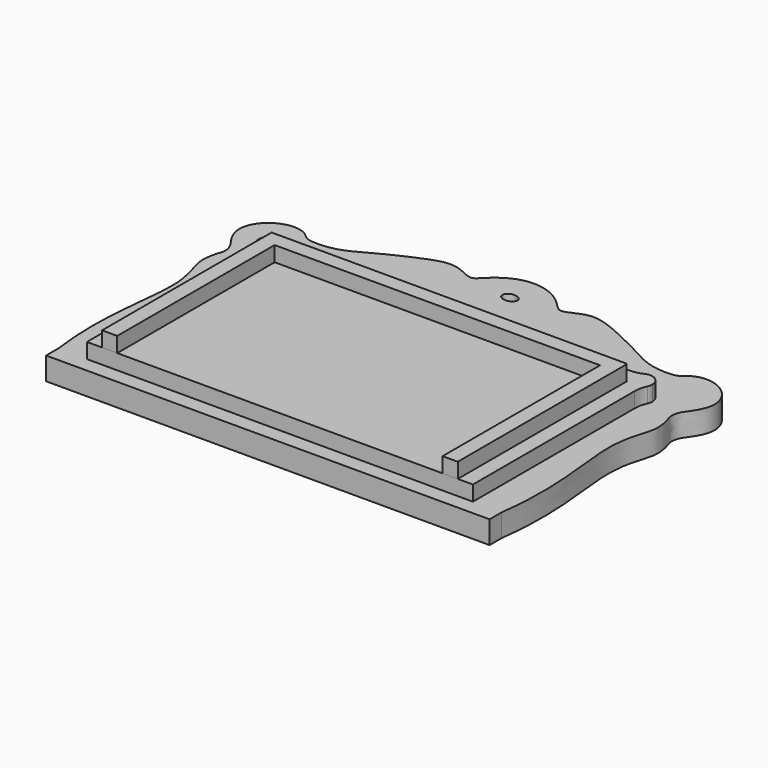
from build123d import *

# Parameters (mm, degrees)
F2_W      = 292.994
F2_H      = 10
F3_DEPTH  = 15
F5_DEPTH  = 10
F6_R      = 20
F8_DEPTH  = 10
F9_W      = 215
F9_H      = 130
F10_DEPTH = 10


# Not quite as in the source:
# - a feature of the source that left no trace in its solid (it failed there, or was rolled back) is left out
# - a feature names something its author has since deleted; it is built from what else it names


with BuildPart() as f3:
    # F2 (on offset) → F3 (new body)
    with BuildSketch(Plane.XY.offset(100)):
        with BuildLine():
            add(Edge.make_bspline(
                [(-146.497, 0), (-149.5984924285, 24.1158641447), (-148.0861706874, 57.3285451295), (-141.9737942158, 98.5465216918), (-150.8716245384, 120.1352309784), (-150.0828583406, 127.8333799004), (-149.2091995607, 133.0357574413), (-146.7644359487, 138.969514697), (-148.7060186985, 145.4416060002), (-153.4320405507, 150.8180485227), (-159.2044434643, 163.229297572), (-152.2232789146, 177.3369452319), (-138.5120912335, 183.3796622376), (-127.657061459, 180.8243319765), (-123.7549340061, 175.7598872143), (-115.4966109213, 174.5749138288), (-101.1868476342, 175.8719474345), (-83.9780063011, 186.2524528593), (-68.1221038647, 193.6100878861), (-57.6143130787, 198.1949467154), (-46.4912789312, 200.9893875839), (-38.3855377787, 198.1650207363), (-34.3252044535, 195.9531038256), (-28.5769681871, 194.0801714579), (-24.8215233637, 198.3952390386), (-15.2356704617, 207.2522812764), (0, 211.4399134414), (15.2356704617, 207.2522812764), (24.8215233637, 198.3952390386), (28.5769681871, 194.0801714579), (34.3252044535, 195.9531038256), (38.3855377787, 198.1650207363), (46.4912789312, 200.9893875839), (57.6143130787, 198.1949467154), (68.1221038647, 193.6100878861), (83.9780063011, 186.2524528593), (101.1868476342, 175.8719474345), (115.4966109213, 174.5749138288), (123.7549340061, 175.7598872143), (127.657061459, 180.8243319765), (138.5120912335, 183.3796622376), (152.2232789146, 177.3369452319), (159.2044434643, 163.229297572), (153.4320405507, 150.8180485227), (148.7060186985, 145.4416060002), (146.7644359487, 138.969514697), (149.2091995607, 133.0357574413), (150.0828583406, 127.8333799004), (150.8716245384, 120.1352309784), (141.9737942158, 98.5465216918), (148.0861706874, 57.3285451295), (149.5984924285, 24.1158641447), (146.497, 0)],
                knots=[0, 0, 0, 0, 0.0445117001, 0.0808774056, 0.107575939, 0.1227793119, 0.1357551155, 0.1500456603, 0.1643362052, 0.1797671231, 0.2002043009, 0.2219477978, 0.2436912948, 0.2620418522, 0.2758571435, 0.2916470183, 0.3132257177, 0.3392061483, 0.3632884541, 0.3827866647, 0.4019539182, 0.4183166408, 0.4309215947, 0.4439460967, 0.456795292, 0.4773590218, 0.5, 0.5226409782, 0.543204708, 0.5560539033, 0.5690784053, 0.5816833592, 0.5980460818, 0.6172133353, 0.6367115459, 0.6607938517, 0.6867742823, 0.7083529817, 0.7241428565, 0.7379581478, 0.7563087052, 0.7780522022, 0.7997956991, 0.8202328769, 0.8356637948, 0.8499543397, 0.8642448845, 0.8772206881, 0.892424061, 0.9191225944, 0.9554882999, 1, 1, 1, 1], degree=3))
            Line((-146.497, 0), (146.497, 0))
        make_face()
        with BuildLine():
            add(Edge.make_bspline(
                [(5, 190), (5, 196.4951905284), (-2.5, 193.2475952642), (-10, 190), (-2.5, 186.7524047358), (5, 183.5048094716), (5, 190)],
                knots=[0, 0, 0, 2.0943951024, 2.0943951024, 4.1887902048, 4.1887902048, 6.2831853072, 6.2831853072, 6.2831853072], degree=2, weights=[1, 0.5, 1, 0.5, 1, 0.5, 1]))
        make_face(mode=Mode.SUBTRACT)
        with Locations((0, -5)):
            Rectangle(F2_W, F2_H)
    extrude(amount=F3_DEPTH)


with BuildPart() as f5:
    # F4 (on face) → F5 (new body)
    with BuildSketch(Plane.XY.offset(115)):
        with BuildLine():
            Line((-116.9098300563, 150), (-127.5, 150))
            Line((-127.5, 150), (-117.5, 140))
            Line((-117.5, 140), (-116.9098300563, 140))
            ThreePointArc((-116.9098300563, 140), (-115.4937073078, 142.3238343267), (-115, 145))
            ThreePointArc((-115, 145), (-115.4937073078, 147.6761656733), (-116.9098300563, 150))
        make_face()
        with BuildLine():
            Line((116.9098300563, 150), (-116.9098300563, 150))
            ThreePointArc((-116.9098300563, 150), (-115.4937073078, 147.6761656733), (-115, 145))
            ThreePointArc((-115, 145), (-115.4937073078, 142.3238343267), (-116.9098300563, 140))
            Line((-116.9098300563, 140), (116.9098300563, 140))
            ThreePointArc((116.9098300563, 140), (115, 145), (116.9098300563, 150))
        make_face()
        with BuildLine():
            Line((117.5, 140), (117.5, 139.4098300563))
            ThreePointArc((117.5, 139.4098300563), (122.5, 137.5), (127.5, 139.4098300563))
            Line((127.5, 139.4098300563), (127.5, 150))
            Line((127.5, 150), (116.9098300563, 150))
            ThreePointArc((116.9098300563, 150), (115, 145), (116.9098300563, 140))
            Line((116.9098300563, 140), (117.5, 140))
        make_face()
        with BuildLine():
            Line((-117.5, 139.4098300563), (-117.5, 0))
            Line((-117.5, 0), (117.5, 0))
            Line((117.5, 0), (117.5, 139.4098300563))
            ThreePointArc((117.5, 139.4098300563), (117.1966991411, 139.6966991411), (116.9098300563, 140))
            Line((116.9098300563, 140), (-116.9098300563, 140))
            ThreePointArc((-116.9098300563, 140), (-117.1966991411, 139.6966991411), (-117.5, 139.4098300563))
        make_face()
        with BuildLine():
            Line((-127.5, 150), (-127.5, 139.4098300563))
            ThreePointArc((-127.5, 139.4098300563), (-122.5, 137.5), (-117.5, 139.4098300563))
            Line((-117.5, 139.4098300563), (-117.5, 140))
            Line((-117.5, 140), (-127.5, 150))
        make_face()
        with BuildLine():
            Line((-117.5, 140), (-117.5, 139.4098300563))
            ThreePointArc((-117.5, 139.4098300563), (-117.1966991411, 139.6966991411), (-116.9098300563, 140))
            Line((-116.9098300563, 140), (-117.5, 140))
        make_face()
        with BuildLine():
            Line((-127.5, 139.4098300563), (-127.5, 0))
            Line((-127.5, 0), (-117.5, 0))
            Line((-117.5, 0), (-117.5, 139.4098300563))
            ThreePointArc((-117.5, 139.4098300563), (-122.5, 137.5), (-127.5, 139.4098300563))
        make_face()
        with BuildLine():
            Line((117.5, 139.4098300563), (117.5, 0))
            Line((117.5, 0), (127.5, 0))
            Line((127.5, 0), (127.5, 139.4098300563))
            ThreePointArc((127.5, 139.4098300563), (122.5, 137.5), (117.5, 139.4098300563))
        make_face()
        with BuildLine():
            ThreePointArc((-116.9098300563, 150), (-127.8033008589, 150.3033008589), (-127.5, 139.4098300563))
            Line((-127.5, 139.4098300563), (-127.5, 150))
            Line((-127.5, 150), (-116.9098300563, 150))
        make_face()
        with BuildLine():
            ThreePointArc((130, 145), (125.1761656733, 152.0062926922), (116.9098300563, 150))
            Line((116.9098300563, 150), (127.5, 150))
            Line((127.5, 150), (127.5, 139.4098300563))
            ThreePointArc((127.5, 139.4098300563), (129.3465319688, 141.9381378215), (130, 145))
        make_face()
    extrude(amount=F5_DEPTH)

    # F6
    f6_edges = [f5.edges().sort_by_distance(p)[0] for p in [
        (-116.90983, 150, 120),
        (-127.5, 139.40983, 120),
        (116.90983, 150, 120),
        (127.5, 139.40983, 120),
    ]]
    fillet(f6_edges, radius=F6_R)


with BuildPart() as f8:
    # F7 (on face) → F8 (new body)
    with BuildSketch(Plane.XY.offset(125)):
        with BuildLine():
            Line((-117.5, 0), (117.5, 0))
            Line((117.5, 0), (117.5, 139.4098300563))
            ThreePointArc((117.5, 139.4098300563), (117.1966991411, 139.6966991411), (116.9098300563, 140))
            Line((116.9098300563, 140), (-117.5, 140))
            Line((-117.5, 140), (-117.5, 0))
        make_face()
    extrude(amount=F8_DEPTH)

    # F9 (on face) → F10 (cut)
    with BuildSketch(Plane.XY.offset(135)):
        with Locations((0, 65)):
            Rectangle(F9_W, F9_H)
    extrude(amount=-F10_DEPTH, mode=Mode.SUBTRACT)


solid = Compound([f3.part, f5.part, f8.part])
